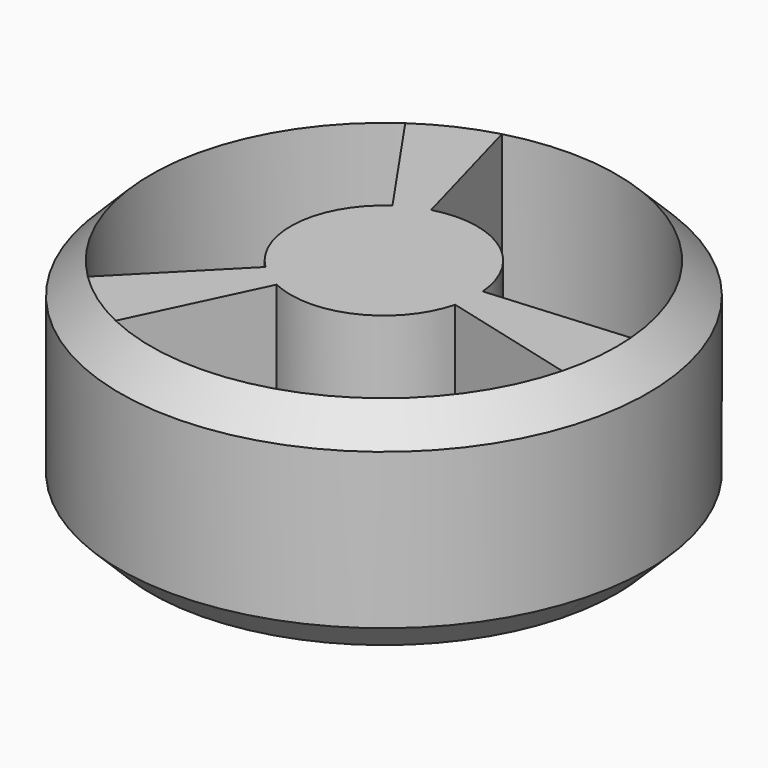
from build123d import *

# Parameters (mm, degrees)
F1_DEPTH = 1
F2_DEPTH = 7
F3_DEPTH = 6
F5_SIZE  = 0.99999


# Not quite as in the source:
# - a fillet or chamfer that OpenCascade refuses, or shapes differently, is made with other operations: its cross-section is extruded or revolved along the edge and cut away or added
# - a fillet or chamfer is up to 0.001 mm smaller than in the source, because OpenCascade refuses the exact size


with BuildPart() as f1:
    # F0 (on Top) → F1 (new body)
    with BuildSketch(Plane.XY):
        with BuildLine():
            ThreePointArc((-3.2217815715, -6.7727485931), (3.1654449772, -6.7992615846), (7.2568170006, -1.8943619029))
            Line((7.2568170006, -1.8943619029), (2.9027268003, -0.7577447612))
            ThreePointArc((2.9027268003, -0.7577447612), (1.2661779909, -2.7197046339), (-1.2887126286, -2.7090994373))
            Line((-1.2887126286, -2.7090994373), (-3.2217815715, -6.7727485931))
        make_face()
        with BuildLine():
            Line((-1.7017926197, 2.4706075932), (-4.2544815494, 6.1765189829))
            ThreePointArc((-4.2544815494, 6.1765189829), (-7.4710557479, 0.6582750278), (-5.2689740322, -5.3374069217))
            Line((-5.2689740322, -5.3374069217), (-2.1075896129, -2.1349627687))
            ThreePointArc((-2.1075896129, -2.1349627687), (-2.9884222991, 0.2633100111), (-1.7017926197, 2.4706075932))
        make_face()
        with BuildLine():
            ThreePointArc((3, 0), (2.9976253723, 0.119340385), (2.9905052483, 0.2384918441))
            Line((2.9905052483, 0.2384918441), (0.9968350828, 0.0794972814))
            ThreePointArc((0.9968350828, 0.0794972814), (0.9992084574, 0.0397801283), (1, 0))
            ThreePointArc((1, 0), (0.9918607765, -0.1273271376), (0.9675756001, -0.2525815871))
            Line((0.9675756001, -0.2525815871), (2.9027268003, -0.7577447612))
            ThreePointArc((2.9027268003, -0.7577447612), (2.9755823296, -0.3819814127), (3, 0))
        make_face()
        with BuildLine():
            Line((-0.7951371874, 2.8927075298), (-1.9878429685, 7.2317688246))
            ThreePointArc((-1.9878429685, 7.2317688246), (-3.1654449772, 6.7992615846), (-4.2544815494, 6.1765189829))
            Line((-4.2544815494, 6.1765189829), (-1.7017926197, 2.4706075932))
            ThreePointArc((-1.7017926197, 2.4706075932), (-1.2661779909, 2.7197046339), (-0.7951371874, 2.8927075298))
        make_face()
        with BuildLine():
            ThreePointArc((-5.2689740322, -5.3374069217), (-4.3056107707, -6.1409865568), (-3.2217815715, -6.7727485931))
            Line((-3.2217815715, -6.7727485931), (-1.2887126286, -2.7090994373))
            ThreePointArc((-1.2887126286, -2.7090994373), (-1.7222443083, -2.4563946227), (-2.1075896129, -2.1349627687))
            Line((-2.1075896129, -2.1349627687), (-5.2689740322, -5.3374069217))
        make_face()
        with BuildLine():
            ThreePointArc((-2.1075896129, -2.1349627687), (-1.7222443083, -2.4563946227), (-1.2887126286, -2.7090994373))
            Line((-1.2887126286, -2.7090994373), (-0.4295708762, -0.9030331458))
            ThreePointArc((-0.4295708762, -0.9030331458), (-0.5740814361, -0.8187982076), (-0.702529871, -0.7116542562))
            Line((-0.702529871, -0.7116542562), (-2.1075896129, -2.1349627687))
        make_face()
        with BuildLine():
            Line((-0.2650457291, 0.9642358433), (-0.7951371874, 2.8927075298))
            ThreePointArc((-0.7951371874, 2.8927075298), (-1.2661779909, 2.7197046339), (-1.7017926197, 2.4706075932))
            Line((-1.7017926197, 2.4706075932), (-0.5672642066, 0.8235358644))
            ThreePointArc((-0.5672642066, 0.8235358644), (-0.4220593303, 0.9065682113), (-0.2650457291, 0.9642358433))
        make_face()
        with BuildLine():
            ThreePointArc((-1.2887126286, -2.7090994373), (1.2661779909, -2.7197046339), (2.9027268003, -0.7577447612))
            Line((2.9027268003, -0.7577447612), (0.9675756001, -0.2525815871))
            ThreePointArc((0.9675756001, -0.2525815871), (0.4220593303, -0.9065682113), (-0.4295708762, -0.9030331458))
            Line((-0.4295708762, -0.9030331458), (-1.2887126286, -2.7090994373))
        make_face()
        with BuildLine():
            Line((-0.5672642066, 0.8235358644), (-1.7017926197, 2.4706075932))
            ThreePointArc((-1.7017926197, 2.4706075932), (-2.9884222991, 0.2633100111), (-2.1075896129, -2.1349627687))
            Line((-2.1075896129, -2.1349627687), (-0.702529871, -0.7116542562))
            ThreePointArc((-0.702529871, -0.7116542562), (-0.9961407664, 0.0877700037), (-0.5672642066, 0.8235358644))
        make_face()
        with BuildLine():
            Line((2.9905052483, 0.2384918441), (7.4762631208, 0.5962296102))
            ThreePointArc((7.4762631208, 0.5962296102), (4.3056107707, 6.1409865568), (-1.9878429685, 7.2317688246))
            Line((-1.9878429685, 7.2317688246), (-0.7951371874, 2.8927075298))
            ThreePointArc((-0.7951371874, 2.8927075298), (1.7222443083, 2.4563946227), (2.9905052483, 0.2384918441))
        make_face()
        with BuildLine():
            Line((0.9968350828, 0.0794972814), (2.9905052483, 0.2384918441))
            ThreePointArc((2.9905052483, 0.2384918441), (1.7222443083, 2.4563946227), (-0.7951371874, 2.8927075298))
            Line((-0.7951371874, 2.8927075298), (-0.2650457291, 0.9642358433))
            ThreePointArc((-0.2650457291, 0.9642358433), (0.5740814361, 0.8187982076), (0.9968350828, 0.0794972814))
        make_face()
        with BuildLine():
            ThreePointArc((7.5, 0), (7.4940634307, 0.2983509626), (7.4762631208, 0.5962296102))
            Line((7.4762631208, 0.5962296102), (2.9905052483, 0.2384918441))
            ThreePointArc((2.9905052483, 0.2384918441), (2.9976253723, 0.119340385), (3, 0))
            ThreePointArc((3, 0), (2.9755823296, -0.3819814127), (2.9027268003, -0.7577447612))
            Line((2.9027268003, -0.7577447612), (7.2568170006, -1.8943619029))
            ThreePointArc((7.2568170006, -1.8943619029), (7.4389558241, -0.9549535316), (7.5, 0))
        make_face()
        with BuildLine():
            Line((7.4762631208, 0.5962296102), (8.4730982036, 0.6757268916))
            ThreePointArc((8.4730982036, 0.6757268916), (4.8796922068, 6.9597847644), (-2.2528886976, 8.1960046679))
            Line((-2.2528886976, 8.1960046679), (-1.9878429685, 7.2317688246))
            ThreePointArc((-1.9878429685, 7.2317688246), (4.3056107707, 6.1409865568), (7.4762631208, 0.5962296102))
        make_face()
        with BuildLine():
            Line((-1.9878429685, 7.2317688246), (-2.2528886976, 8.1960046679))
            ThreePointArc((-2.2528886976, 8.1960046679), (-3.5875043075, 7.7058297959), (-4.821745756, 7.0000548473))
            Line((-4.821745756, 7.0000548473), (-4.2544815494, 6.1765189829))
            ThreePointArc((-4.2544815494, 6.1765189829), (-3.1654449772, 6.7992615846), (-1.9878429685, 7.2317688246))
        make_face()
        with BuildLine():
            Line((-4.2544815494, 6.1765189829), (-4.821745756, 7.0000548473))
            ThreePointArc((-4.821745756, 7.0000548473), (-8.4671965143, 0.7460450315), (-5.9715039032, -6.049061178))
            Line((-5.9715039032, -6.049061178), (-5.2689740322, -5.3374069217))
            ThreePointArc((-5.2689740322, -5.3374069217), (-7.4710557479, 0.6582750278), (-4.2544815494, 6.1765189829))
        make_face()
        with BuildLine():
            ThreePointArc((-5.9715039032, -6.049061178), (-4.8796922068, -6.9597847644), (-3.6513524477, -7.6757817389))
            Line((-3.6513524477, -7.6757817389), (-3.2217815715, -6.7727485931))
            ThreePointArc((-3.2217815715, -6.7727485931), (-4.3056107707, -6.1409865568), (-5.2689740322, -5.3374069217))
            Line((-5.2689740322, -5.3374069217), (-5.9715039032, -6.049061178))
        make_face()
        with BuildLine():
            ThreePointArc((-3.6513524477, -7.6757817389), (3.5875043075, -7.7058297959), (8.2243926007, -2.14694349))
            Line((8.2243926007, -2.14694349), (7.2568170006, -1.8943619029))
            ThreePointArc((7.2568170006, -1.8943619029), (3.1654449772, -6.7992615846), (-3.2217815715, -6.7727485931))
            Line((-3.2217815715, -6.7727485931), (-3.6513524477, -7.6757817389))
        make_face()
        with BuildLine():
            ThreePointArc((8.2243926007, -2.14694349), (8.4308166006, -1.0822806692), (8.5, 0))
            ThreePointArc((8.5, 0), (8.4932718881, 0.338131091), (8.4730982036, 0.6757268916))
            Line((8.4730982036, 0.6757268916), (7.4762631208, 0.5962296102))
            ThreePointArc((7.4762631208, 0.5962296102), (7.4940634307, 0.2983509626), (7.5, 0))
            ThreePointArc((7.5, 0), (7.4389558241, -0.9549535316), (7.2568170006, -1.8943619029))
            Line((7.2568170006, -1.8943619029), (8.2243926007, -2.14694349))
        make_face()
    extrude(amount=F1_DEPTH)

    # F0 (on Top) → F2 (join)
    with BuildSketch(Plane.XY):
        with BuildLine():
            Line((-4.2544815494, 6.1765189829), (-4.821745756, 7.0000548473))
            ThreePointArc((-4.821745756, 7.0000548473), (-8.4671965143, 0.7460450315), (-5.9715039032, -6.049061178))
            Line((-5.9715039032, -6.049061178), (-5.2689740322, -5.3374069217))
            ThreePointArc((-5.2689740322, -5.3374069217), (-7.4710557479, 0.6582750278), (-4.2544815494, 6.1765189829))
        make_face()
        with BuildLine():
            ThreePointArc((-5.9715039032, -6.049061178), (-4.8796922068, -6.9597847644), (-3.6513524477, -7.6757817389))
            Line((-3.6513524477, -7.6757817389), (-3.2217815715, -6.7727485931))
            ThreePointArc((-3.2217815715, -6.7727485931), (-4.3056107707, -6.1409865568), (-5.2689740322, -5.3374069217))
            Line((-5.2689740322, -5.3374069217), (-5.9715039032, -6.049061178))
        make_face()
        with BuildLine():
            ThreePointArc((-3.6513524477, -7.6757817389), (3.5875043075, -7.7058297959), (8.2243926007, -2.14694349))
            Line((8.2243926007, -2.14694349), (7.2568170006, -1.8943619029))
            ThreePointArc((7.2568170006, -1.8943619029), (3.1654449772, -6.7992615846), (-3.2217815715, -6.7727485931))
            Line((-3.2217815715, -6.7727485931), (-3.6513524477, -7.6757817389))
        make_face()
        with BuildLine():
            ThreePointArc((8.2243926007, -2.14694349), (8.4308166006, -1.0822806692), (8.5, 0))
            ThreePointArc((8.5, 0), (8.4932718881, 0.338131091), (8.4730982036, 0.6757268916))
            Line((8.4730982036, 0.6757268916), (7.4762631208, 0.5962296102))
            ThreePointArc((7.4762631208, 0.5962296102), (7.4940634307, 0.2983509626), (7.5, 0))
            ThreePointArc((7.5, 0), (7.4389558241, -0.9549535316), (7.2568170006, -1.8943619029))
            Line((7.2568170006, -1.8943619029), (8.2243926007, -2.14694349))
        make_face()
        with BuildLine():
            Line((7.4762631208, 0.5962296102), (8.4730982036, 0.6757268916))
            ThreePointArc((8.4730982036, 0.6757268916), (4.8796922068, 6.9597847644), (-2.2528886976, 8.1960046679))
            Line((-2.2528886976, 8.1960046679), (-1.9878429685, 7.2317688246))
            ThreePointArc((-1.9878429685, 7.2317688246), (4.3056107707, 6.1409865568), (7.4762631208, 0.5962296102))
        make_face()
        with BuildLine():
            Line((-1.9878429685, 7.2317688246), (-2.2528886976, 8.1960046679))
            ThreePointArc((-2.2528886976, 8.1960046679), (-3.5875043075, 7.7058297959), (-4.821745756, 7.0000548473))
            Line((-4.821745756, 7.0000548473), (-4.2544815494, 6.1765189829))
            ThreePointArc((-4.2544815494, 6.1765189829), (-3.1654449772, 6.7992615846), (-1.9878429685, 7.2317688246))
        make_face()
        with BuildLine():
            Line((-0.2650457291, 0.9642358433), (-0.7951371874, 2.8927075298))
            ThreePointArc((-0.7951371874, 2.8927075298), (-1.2661779909, 2.7197046339), (-1.7017926197, 2.4706075932))
            Line((-1.7017926197, 2.4706075932), (-0.5672642066, 0.8235358644))
            ThreePointArc((-0.5672642066, 0.8235358644), (-0.4220593303, 0.9065682113), (-0.2650457291, 0.9642358433))
        make_face()
        with BuildLine():
            Line((-0.5672642066, 0.8235358644), (-1.7017926197, 2.4706075932))
            ThreePointArc((-1.7017926197, 2.4706075932), (-2.9884222991, 0.2633100111), (-2.1075896129, -2.1349627687))
            Line((-2.1075896129, -2.1349627687), (-0.702529871, -0.7116542562))
            ThreePointArc((-0.702529871, -0.7116542562), (-0.9961407664, 0.0877700037), (-0.5672642066, 0.8235358644))
        make_face()
        with BuildLine():
            ThreePointArc((-2.1075896129, -2.1349627687), (-1.7222443083, -2.4563946227), (-1.2887126286, -2.7090994373))
            Line((-1.2887126286, -2.7090994373), (-0.4295708762, -0.9030331458))
            ThreePointArc((-0.4295708762, -0.9030331458), (-0.5740814361, -0.8187982076), (-0.702529871, -0.7116542562))
            Line((-0.702529871, -0.7116542562), (-2.1075896129, -2.1349627687))
        make_face()
        with BuildLine():
            ThreePointArc((-1.2887126286, -2.7090994373), (1.2661779909, -2.7197046339), (2.9027268003, -0.7577447612))
            Line((2.9027268003, -0.7577447612), (0.9675756001, -0.2525815871))
            ThreePointArc((0.9675756001, -0.2525815871), (0.4220593303, -0.9065682113), (-0.4295708762, -0.9030331458))
            Line((-0.4295708762, -0.9030331458), (-1.2887126286, -2.7090994373))
        make_face()
        with BuildLine():
            ThreePointArc((3, 0), (2.9976253723, 0.119340385), (2.9905052483, 0.2384918441))
            Line((2.9905052483, 0.2384918441), (0.9968350828, 0.0794972814))
            ThreePointArc((0.9968350828, 0.0794972814), (0.9992084574, 0.0397801283), (1, 0))
            ThreePointArc((1, 0), (0.9918607765, -0.1273271376), (0.9675756001, -0.2525815871))
            Line((0.9675756001, -0.2525815871), (2.9027268003, -0.7577447612))
            ThreePointArc((2.9027268003, -0.7577447612), (2.9755823296, -0.3819814127), (3, 0))
        make_face()
        with BuildLine():
            Line((0.9968350828, 0.0794972814), (2.9905052483, 0.2384918441))
            ThreePointArc((2.9905052483, 0.2384918441), (1.7222443083, 2.4563946227), (-0.7951371874, 2.8927075298))
            Line((-0.7951371874, 2.8927075298), (-0.2650457291, 0.9642358433))
            ThreePointArc((-0.2650457291, 0.9642358433), (0.5740814361, 0.8187982076), (0.9968350828, 0.0794972814))
        make_face()
        with BuildLine():
            Line((-0.7951371874, 2.8927075298), (-1.9878429685, 7.2317688246))
            ThreePointArc((-1.9878429685, 7.2317688246), (-3.1654449772, 6.7992615846), (-4.2544815494, 6.1765189829))
            Line((-4.2544815494, 6.1765189829), (-1.7017926197, 2.4706075932))
            ThreePointArc((-1.7017926197, 2.4706075932), (-1.2661779909, 2.7197046339), (-0.7951371874, 2.8927075298))
        make_face()
        with BuildLine():
            ThreePointArc((-5.2689740322, -5.3374069217), (-4.3056107707, -6.1409865568), (-3.2217815715, -6.7727485931))
            Line((-3.2217815715, -6.7727485931), (-1.2887126286, -2.7090994373))
            ThreePointArc((-1.2887126286, -2.7090994373), (-1.7222443083, -2.4563946227), (-2.1075896129, -2.1349627687))
            Line((-2.1075896129, -2.1349627687), (-5.2689740322, -5.3374069217))
        make_face()
        with BuildLine():
            ThreePointArc((7.5, 0), (7.4940634307, 0.2983509626), (7.4762631208, 0.5962296102))
            Line((7.4762631208, 0.5962296102), (2.9905052483, 0.2384918441))
            ThreePointArc((2.9905052483, 0.2384918441), (2.9976253723, 0.119340385), (3, 0))
            ThreePointArc((3, 0), (2.9755823296, -0.3819814127), (2.9027268003, -0.7577447612))
            Line((2.9027268003, -0.7577447612), (7.2568170006, -1.8943619029))
            ThreePointArc((7.2568170006, -1.8943619029), (7.4389558241, -0.9549535316), (7.5, 0))
        make_face()
        with BuildLine():
            Line((0, 0), (-0.2650457291, 0.9642358433))
            ThreePointArc((-0.2650457291, 0.9642358433), (-0.4220593303, 0.9065682113), (-0.5672642066, 0.8235358644))
            Line((-0.5672642066, 0.8235358644), (0, 0))
        make_face()
        with BuildLine():
            Line((-0.702529871, -0.7116542562), (0, 0))
            Line((0, 0), (-0.5672642066, 0.8235358644))
            ThreePointArc((-0.5672642066, 0.8235358644), (-0.9961407664, 0.0877700037), (-0.702529871, -0.7116542562))
        make_face()
        with BuildLine():
            Line((-0.4295708762, -0.9030331458), (0, 0))
            Line((0, 0), (-0.702529871, -0.7116542562))
            ThreePointArc((-0.702529871, -0.7116542562), (-0.5740814361, -0.8187982076), (-0.4295708762, -0.9030331458))
        make_face()
        with BuildLine():
            ThreePointArc((-0.4295708762, -0.9030331458), (0.4220593303, -0.9065682113), (0.9675756001, -0.2525815871))
            Line((0.9675756001, -0.2525815871), (0, 0))
            Line((0, 0), (-0.4295708762, -0.9030331458))
        make_face()
        with BuildLine():
            ThreePointArc((1, 0), (0.9992084574, 0.0397801283), (0.9968350828, 0.0794972814))
            Line((0.9968350828, 0.0794972814), (0, 0))
            Line((0, 0), (0.9675756001, -0.2525815871))
            ThreePointArc((0.9675756001, -0.2525815871), (0.9918607765, -0.1273271376), (1, 0))
        make_face()
        with BuildLine():
            Line((0, 0), (0.9968350828, 0.0794972814))
            ThreePointArc((0.9968350828, 0.0794972814), (0.5740814361, 0.8187982076), (-0.2650457291, 0.9642358433))
            Line((-0.2650457291, 0.9642358433), (0, 0))
        make_face()
    extrude(amount=F2_DEPTH)

    # F0 (on Top) → F3 (cut)
    with BuildSketch(Plane.XY):
        with BuildLine():
            ThreePointArc((-0.4295708762, -0.9030331458), (0.4220593303, -0.9065682113), (0.9675756001, -0.2525815871))
            Line((0.9675756001, -0.2525815871), (0, 0))
            Line((0, 0), (-0.4295708762, -0.9030331458))
        make_face()
        with BuildLine():
            ThreePointArc((1, 0), (0.9992084574, 0.0397801283), (0.9968350828, 0.0794972814))
            Line((0.9968350828, 0.0794972814), (0, 0))
            Line((0, 0), (0.9675756001, -0.2525815871))
            ThreePointArc((0.9675756001, -0.2525815871), (0.9918607765, -0.1273271376), (1, 0))
        make_face()
        with BuildLine():
            Line((0, 0), (0.9968350828, 0.0794972814))
            ThreePointArc((0.9968350828, 0.0794972814), (0.5740814361, 0.8187982076), (-0.2650457291, 0.9642358433))
            Line((-0.2650457291, 0.9642358433), (0, 0))
        make_face()
        with BuildLine():
            Line((-0.702529871, -0.7116542562), (0, 0))
            Line((0, 0), (-0.5672642066, 0.8235358644))
            ThreePointArc((-0.5672642066, 0.8235358644), (-0.9961407664, 0.0877700037), (-0.702529871, -0.7116542562))
        make_face()
        with BuildLine():
            Line((-0.4295708762, -0.9030331458), (0, 0))
            Line((0, 0), (-0.702529871, -0.7116542562))
            ThreePointArc((-0.702529871, -0.7116542562), (-0.5740814361, -0.8187982076), (-0.4295708762, -0.9030331458))
        make_face()
        with BuildLine():
            Line((0, 0), (-0.2650457291, 0.9642358433))
            ThreePointArc((-0.2650457291, 0.9642358433), (-0.4220593303, 0.9065682113), (-0.5672642066, 0.8235358644))
            Line((-0.5672642066, 0.8235358644), (0, 0))
        make_face()
    extrude(amount=F3_DEPTH, mode=Mode.SUBTRACT)

    # F4: chamfer of 1 on 1 edges, made by hand

    # F4_s1 → F4_t2 (revolve, cut)
    with BuildSketch(Plane(origin=(0, 0, 0), x_dir=(0, 0, 1), z_dir=(0.9642358433, 0.2650457291, 0))):
        Polygon((6, -8.5), (7, -7.5), (7, -8.5), align=None)
    revolve(axis=Axis((0, 0, 7), (0, 0, 1)), mode=Mode.SUBTRACT)

    # F5 (size 1 in the source; OpenCascade refuses exactly that, so slightly less here)
    f5_edges = [f1.edges().sort_by_distance(p)[0] for p in [
        (-8.224393, 2.146943, 0),
    ]]
    chamfer(f5_edges, length=F5_SIZE)


solid = f1.part
